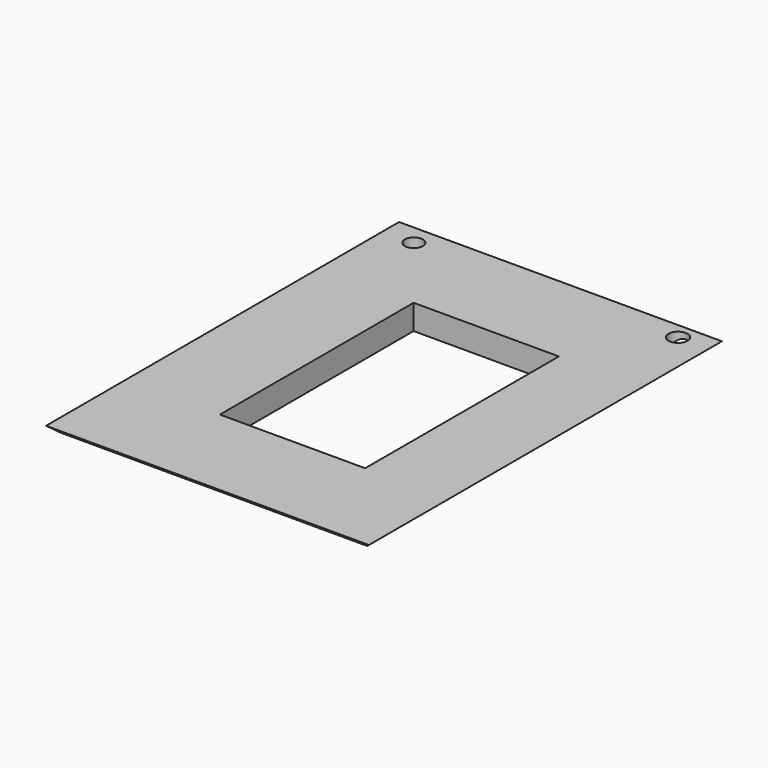
from build123d import *

# Parameters (mm, degrees)
F0_W        = 69.0733827651
F0_H        = 94.4002903998
F0_R        = 1.9306579711
F0_W_2      = 31.083021313
F0_H_2      = 51.8050361425
F0_R_2      = 2.0350948247
F1_DEPTH    = 5.334
F2_T1_DEPTH = 136.319889095
F2_T3_DEPTH = 161.6467967298


# Not quite as in the source:
# - a fillet or chamfer that OpenCascade refuses, or shapes differently, is made with other operations: its cross-section is extruded or revolved along the edge and cut away or added


with BuildPart() as f1:
    # F0 (on Top) → F1 (new body)
    with BuildSketch(Plane.XY):
        with Locations((1.8707383424, -0.7195156068)):
            Rectangle(F0_W, F0_H)
        with Locations((-26.0464213789, 42.1635434031)):
            Circle(F0_R, mode=Mode.SUBTRACT)
        with Locations((3.021961078, -0.7195146754)):
            Rectangle(F0_W_2, F0_H_2, mode=Mode.SUBTRACT)
        with Locations((29.7878980637, 43.0269613862)):
            Circle(F0_R_2, mode=Mode.SUBTRACT)
    extrude(amount=F1_DEPTH)

    # F2: fillet of radius 19.622727835 on 4 edges, made by hand

    # F2_s2 → F2_t1 (cut)
    with BuildSketch(Plane.YZ.offset(-66.2892062051)):
        with BuildLine():
            ThreePointArc((46.4806295931, 5.334), (40.2655397656, 1.3821787054), (33.0313283271, 0))
            Line((33.0313283271, 0), (46.4806295931, 0))
            Line((46.4806295931, 0), (46.4806295931, 5.334))
        make_face()
        with BuildLine():
            ThreePointArc((-47.9196608067, 5.334), (-41.7045709791, 1.3821787054), (-34.4703595407, 0))
            Line((-34.4703595407, 0), (-47.9196608067, 0))
            Line((-47.9196608067, 0), (-47.9196608067, 5.334))
        make_face()
    extrude(amount=F2_T1_DEPTH, mode=Mode.SUBTRACT)

    # F2_s4 → F2_t3 (cut)
    with BuildSketch(Plane.XZ.offset(-80.1038827581)):
        with BuildLine():
            ThreePointArc((36.4074297249, 5.334), (30.1923398974, 1.3821787054), (22.9581284589, 0))
            Line((22.9581284589, 0), (36.4074297249, 0))
            Line((36.4074297249, 0), (36.4074297249, 5.334))
        make_face()
        with BuildLine():
            ThreePointArc((-32.6659530401, 5.334), (-26.4508632126, 1.3821787054), (-19.2166517741, 0))
            Line((-19.2166517741, 0), (-32.6659530401, 0))
            Line((-32.6659530401, 0), (-32.6659530401, 5.334))
        make_face()
    extrude(amount=F2_T3_DEPTH, mode=Mode.SUBTRACT)


solid = f1.part
